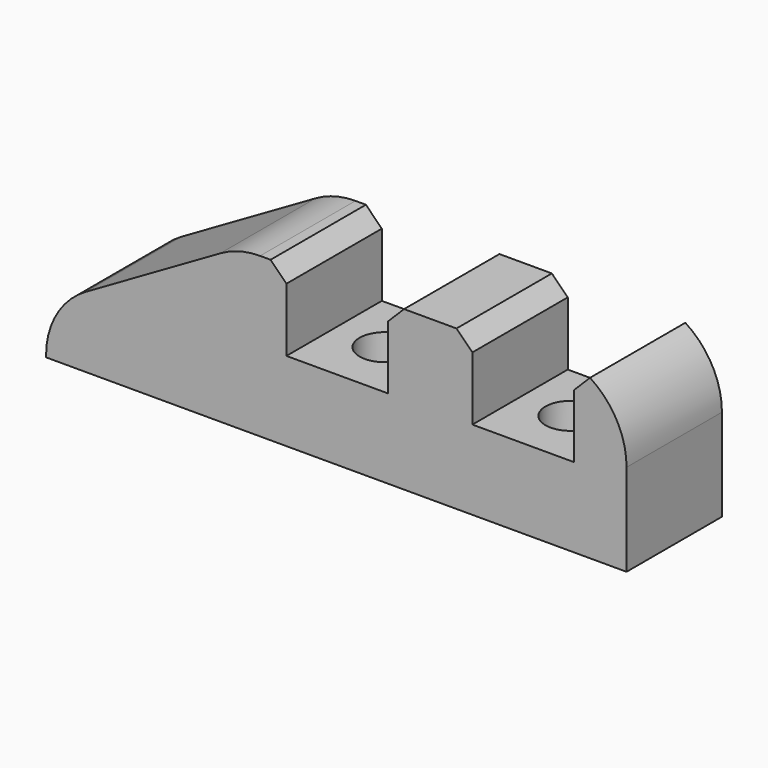
from build123d import *

# Parameters (mm, degrees)
F1_DEPTH     = 7.5
F2_R         = 1.6
F3_DEPTH     = 5.001
F4_R         = 2.75
F4_R_2       = 1.6
F5_DEPTH     = 3.2
F6_R         = 5
F7_SIZE      = 1
F8_DEPTH     = 12
F9_W         = 6.4
F9_H         = 5
F10_DEPTH    = 7.501
F11_SIZE     = 1
F12_T1_DEPTH = 28.5416254125
F13_R        = 1.6
F14_DEPTH    = 5.001
F15_R        = 2.75
F15_R_2      = 1.6
F16_DEPTH    = 3


# Not quite as in the source:
# - a fillet or chamfer that OpenCascade refuses, or shapes differently, is made with other operations: its cross-section is extruded or revolved along the edge and cut away or added


with BuildPart() as f1:
    # F0 (on Front) → F1 (new body)
    with BuildSketch(Plane.XZ):
        Polygon((-24.524355653, 0), (0, 0), (0, 10), (-3, 10), (-3, 5), (-9.4, 5), (-9.4, 10), (-12.4, 10), (-24.524355653, 3), align=None)
    extrude(amount=F1_DEPTH)

    # F2 (on face) → F3 (cut, through all)
    with BuildSketch(Plane.XY.offset(5)):
        with Locations((-6.2, -3.75)):
            Circle(F2_R)
    extrude(amount=-F3_DEPTH, mode=Mode.SUBTRACT)

    # F4 (on face) → F5 (cut)
    with BuildSketch(Plane(origin=(0, 0, 0), x_dir=(1, 0, 0), z_dir=(0, 0, -1))):
        with Locations((-6.2, 3.75)):
            Circle(F4_R)
        with Locations((-6.2, 3.75)):
            Circle(F4_R_2, mode=Mode.SUBTRACT)
    extrude(amount=-F5_DEPTH, mode=Mode.SUBTRACT)

    # F6
    f6_edges = [f1.edges().sort_by_distance(p)[0] for p in [
        (-12.4, -3.75, 10),
        (-24.524356, -3.75, 3),
    ]]
    fillet(f6_edges, radius=F6_R)

    # F7
    f7_edges = [f1.edges().sort_by_distance(p)[0] for p in [
        (-9.4, -3.75, 10),
        (-3, -3.75, 10),
    ]]
    chamfer(f7_edges, length=F7_SIZE)

    # F8 (add): a face of the model
    f8_faces = [f1.faces().sort_by_distance(p)[0] for p in [
        (0, -3.75, 5),
    ]]
    extrude(f8_faces, amount=F8_DEPTH)

    # F9 (on face) → F10 (cut, through all)
    with BuildSketch(Plane.XZ.offset(7.5)):
        with Locations((5.5, 7.5)):
            Rectangle(F9_W, F9_H)
    extrude(amount=-F10_DEPTH, mode=Mode.SUBTRACT)

    # F11
    f11_edges = [f1.edges().sort_by_distance(p)[0] for p in [
        (2.3, -3.75, 10),
        (8.7, -3.75, 10),
    ]]
    chamfer(f11_edges, length=F11_SIZE)

    # F12: fillet of radius 5 on 1 edges, made by hand

    # F12_s2 → F12_t1 (cut)
    with BuildSketch(Plane.XZ.offset(-10.5208127063)):
        with BuildLine():
            ThreePointArc((9.7, 10), (11.3874821937, 8.1895906792), (12, 5.7916749175))
            Line((12, 5.7916749175), (12, 10))
            Line((12, 10), (9.7, 10))
        make_face()
    extrude(amount=F12_T1_DEPTH, mode=Mode.SUBTRACT)

    # F13 (on face) → F14 (cut, through all)
    with BuildSketch(Plane.XY.offset(5)):
        with Locations((5.5, -3.75)):
            Circle(F13_R)
    extrude(amount=-F14_DEPTH, mode=Mode.SUBTRACT)

    # F15 (on face) → F16 (cut)
    with BuildSketch(Plane(origin=(0, 0, 0), x_dir=(1, 0, 0), z_dir=(0, 0, -1))):
        with Locations((5.5, 3.75)):
            Circle(F15_R)
        with Locations((5.5, 3.75)):
            Circle(F15_R_2, mode=Mode.SUBTRACT)
    extrude(amount=-F16_DEPTH, mode=Mode.SUBTRACT)


solid = f1.part
